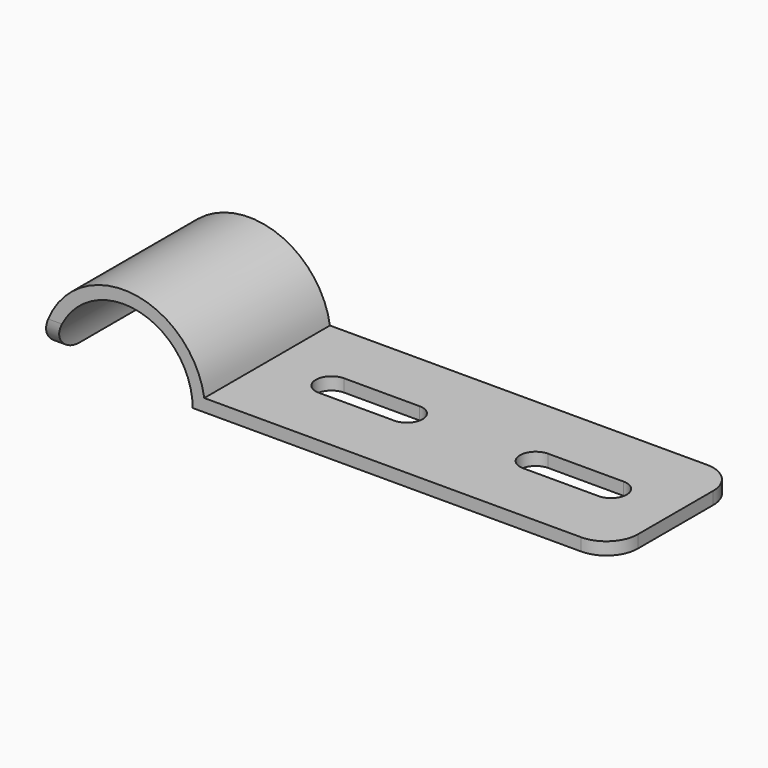
from build123d import *

# Parameters (mm, degrees)
F1_DEPTH = 12.5
F3_DEPTH = 25
F4_R     = 5


# Not quite as in the source:
# - ends of sketch curves that miss each other by under 0.0002 mm in the source are joined


with BuildPart() as f1:
    # F0 (on Front) → F1 (new body, symmetric)
    with BuildSketch(Plane.XZ):
        with BuildLine():
            Line((-33.4226162893, 0), (33.4226162893, 0))
            Line((33.4226162893, 0), (33.4226162893, 2))
            Line((33.4226162893, 2), (-31.5773837107, 2))
            ThreePointArc((-31.5773837107, 2), (-45.4256059397, 12.9612503934), (-57.4226162893, 0))
            Line((-57.4226162893, 0), (-55.4226162893, 0))
            ThreePointArc((-55.4226162893, 0), (-44.4226162893, 11), (-33.4226162893, 0))
        make_face()
    extrude(amount=F1_DEPTH, both=True)

    # F2 (on face) → F3 (cut)
    with BuildSketch(Plane.XY.offset(2)):
        with BuildLine():
            Line((17.172143635, 2.5), (11.172143635, 2.5))
            ThreePointArc((11.172143635, 2.5), (8.6730891224, -0.0009453085), (11.1740342522, -2.4999998213))
            Line((11.1740342522, -2.4999998213), (17.1730889436, -2.5))
            Line((17.1730889436, -2.5), (17.172143635, 2.5))
        make_face()
        with BuildLine():
            Line((23.172143635, 2.5), (17.172143635, 2.5))
            Line((17.172143635, 2.5), (17.1730889436, -2.5))
            Line((17.1730889436, -2.5), (23.172143635, -2.5))
            ThreePointArc((23.172143635, -2.5), (25.672143635, 0), (23.172143635, 2.5))
        make_face()
        with BuildLine():
            ThreePointArc((-9.3288016735, -2.4999998213), (-6.8278565437, -0.0009453085), (-9.3269110564, 2.4999998213))
            Line((-9.3269110564, 2.4999998213), (-21.3269110564, 2.5))
            ThreePointArc((-21.3269110564, 2.5), (-23.8269110564, 0), (-21.3269110564, -2.5))
            Line((-21.3269110564, -2.5), (-9.3288016735, -2.4999998213))
        make_face()
    extrude(amount=-F3_DEPTH, mode=Mode.SUBTRACT)

    # F4
    f4_edges = [f1.edges().sort_by_distance(p)[0] for p in [
        (33.422616, 12.5, 1),
        (33.422616, -12.5, 1),
        (-56.422616, -12.5, 0),
        (-56.422616, 12.5, 0),
    ]]
    fillet(f4_edges, radius=F4_R)


solid = f1.part
